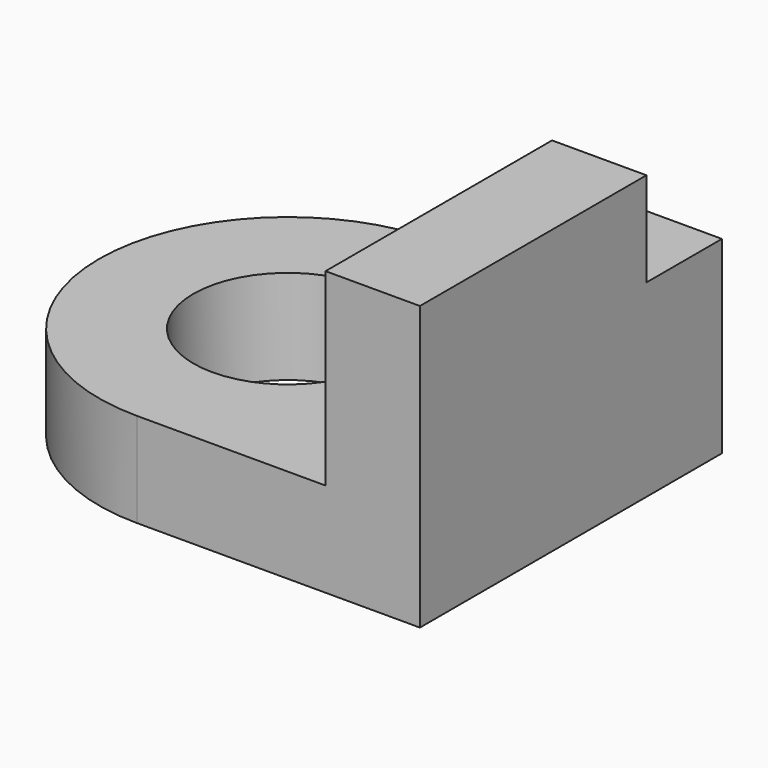
from build123d import *

# Parameters (mm, degrees)
F1_DEPTH = 12.7
F2_DEPTH = 12.7
F3_W     = 12.7
F3_H     = 50.8
F4_DEPTH = 25.4
F5_W     = 12.7
F5_H     = 12.7
F6_DEPTH = 12.7


with BuildPart() as f1:
    # F0 (on Top) → F1 (new body)
    with BuildSketch(Plane.XY):
        with BuildLine():
            ThreePointArc((0, 25.4), (17.9605122421, 17.9605122421), (25.4, 0))
            ThreePointArc((25.4, 0), (17.9605122421, -17.9605122421), (0, -25.4))
            Line((0, -25.4), (38.1, -25.4))
            Line((38.1, -25.4), (38.1, 25.4))
            Line((38.1, 25.4), (0, 25.4))
        make_face()
    extrude(amount=F1_DEPTH)

    # F0 (on Top) → F2 (join)
    with BuildSketch(Plane.XY):
        with BuildLine():
            ThreePointArc((0, -25.4), (17.9605122421, -17.9605122421), (25.4, 0))
            ThreePointArc((25.4, 0), (17.9605122421, 17.9605122421), (0, 25.4))
            Line((0, 25.4), (0, 12.7))
            ThreePointArc((0, 12.7), (8.9802561211, 8.9802561211), (12.7, 0))
            ThreePointArc((12.7, 0), (8.9802561211, -8.9802561211), (0, -12.7))
            Line((0, -12.7), (0, -25.4))
        make_face()
        with BuildLine():
            ThreePointArc((0, 25.4), (17.9605122421, 17.9605122421), (25.4, 0))
            ThreePointArc((25.4, 0), (17.9605122421, -17.9605122421), (0, -25.4))
            Line((0, -25.4), (38.1, -25.4))
            Line((38.1, -25.4), (38.1, 25.4))
            Line((38.1, 25.4), (0, 25.4))
        make_face()
        with BuildLine():
            Line((0, 12.7), (0, 25.4))
            ThreePointArc((0, 25.4), (-25.4, 0), (0, -25.4))
            Line((0, -25.4), (0, -12.7))
            ThreePointArc((0, -12.7), (-12.7, 0), (0, 12.7))
        make_face()
    extrude(amount=F2_DEPTH)

    # F3 (on face) → F4 (join)
    with BuildSketch(Plane.XY.offset(12.7)):
        with Locations((31.75, 0)):
            Rectangle(F3_W, F3_H)
    extrude(amount=F4_DEPTH)

    # F5 (on face) → F6 (cut)
    with BuildSketch(Plane.XY.offset(38.1)):
        with Locations((31.75, 19.05)):
            Rectangle(F5_W, F5_H)
    extrude(amount=-F6_DEPTH, mode=Mode.SUBTRACT)


solid = f1.part
